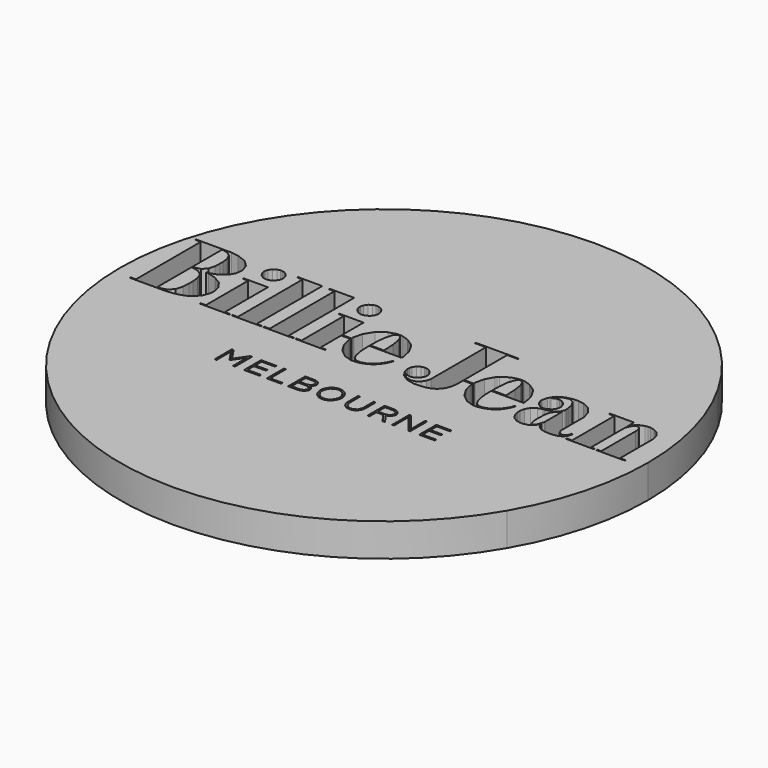
from build123d import *
from build123d import SkipClean  # not in build123d's __all__

# Parameters (mm, degrees)
F1_DEPTH = 5
F3_DEPTH = 50
F5_DEPTH = 25


with BuildPart() as f1:
    # F0 (on Top) → F1 (new body)
    with BuildSketch(Plane.XY):
        with BuildLine():
            Line((34.6410161514, -20), (40, -20))
            Line((40, -20), (40, 0))
            ThreePointArc((40, 0), (38.6370330516, -10.3527618041), (34.6410161514, -20))
        make_face()
        with BuildLine():
            ThreePointArc((-34.6410161514, -20), (0, -40), (34.6410161514, -20))
            Line((34.6410161514, -20), (-34.6410161514, -20))
        make_face()
        with BuildLine():
            Line((-34.6410161514, -20), (34.6410161514, -20))
            ThreePointArc((34.6410161514, -20), (38.6370330516, -10.3527618041), (40, 0))
            ThreePointArc((40, 0), (38.6370330516, 10.3527618041), (34.6410161514, 20))
            Line((34.6410161514, 20), (-34.6410161514, 20))
            ThreePointArc((-34.6410161514, 20), (-38.6370330532, 10.352761798), (-40, -1.26e-08))
            ThreePointArc((-40, -1.26e-08), (-38.6370330499, -10.3527618102), (-34.6410161514, -20))
        make_face()
        with BuildLine():
            ThreePointArc((34.6410161514, 20), (38.6370330516, 10.3527618041), (40, 0))
            Line((40, 0), (40, 20))
            Line((40, 20), (34.6410161514, 20))
        make_face()
        with BuildLine():
            Line((-40, -20), (-34.6410161514, -20))
            ThreePointArc((-34.6410161514, -20), (-38.6370330499, -10.3527618102), (-40, -1.26e-08))
            Line((-40, -1.26e-08), (-40, -20))
        make_face()
        with BuildLine():
            Line((-34.6410161514, 20), (34.6410161514, 20))
            ThreePointArc((34.6410161514, 20), (0, 40), (-34.6410161514, 20))
        make_face()
        with BuildLine():
            Line((-40, 20), (-40, -1.26e-08))
            ThreePointArc((-40, -1.26e-08), (-38.6370330532, 10.352761798), (-34.6410161514, 20))
            Line((-34.6410161514, 20), (-40, 20))
        make_face()
    extrude(amount=F1_DEPTH)

    # F2 (on face) → F3 (cut)
    with BuildSketch(Plane.XY.offset(5)):
        Polygon((-30.8900436095, 5.3960228478), (-31.2979021822, 5.4461403697), (-30.9122151654, 5.5068806273), (-29.7861507128, 5.9029180019), (-28.8714514615, 6.6135517779), (-28.4207478551, 7.4603744723), (-28.2995941933, 8.1075442124), (-28.2995941933, 8.3219055699), (-28.2995941933, 8.6691873117), (-28.6749036146, 9.7093982701), (-29.6517050126, 10.6270392021), (-31.0141661897, 11.1355686232), (-32.1609313579, 11.2905516123), (-32.5421786159, 11.2905516123), (-37.5014980781, 11.2905516123), (-37.5014980781, 11.1399266686), (-36.6901934536, 11.1399266686), (-36.6901934536, -1.1312668693), (-37.5014980781, -1.1312668693), (-37.5014980781, -1.2834716044), (-32.3973553202, -1.2834716044), (-32.2407108263, -1.2834716044), (-31.7707773446, -1.2598292082), (-30.9846131944, -1.1682013039), (-30.120167654, -0.9687117763), (-29.4625658428, -0.7293188956), (-29.255667638, -0.6243989529), (-28.9704608052, -0.4766339765), (-27.9685734084, 0.5046071803), (-27.5370452016, 1.7119219416), (-27.5370452016, 2.1138699153), (-27.5370452016, 2.4286297434), (-27.7838467595, 3.3729092277), (-28.5079087629, 4.3600609836), (-29.687168607, 5.0574571967), align=None)
        Polygon((-33.4731388241, -1.1194456712), (-33.4731388241, 5.3486291042), (-33.1716982722, 5.347267215), (-32.2687657434, 5.1462523715), (-31.5506143391, 4.5683755531), (-31.2033325973, 3.6329755862), (-31.1132027711, 2.6739059853), (-31.1132027711, 2.3532627959), (-31.1132027711, 1.9926617779), (-31.173779602, 0.9080259943), (-31.4693367927, -0.1810495481), (-32.1771923147, -0.8697296704), (-33.1495267163, -1.1164767527), align=None, mode=Mode.SUBTRACT)
        Polygon((-33.1864611509, 5.5275813429), (-33.4731388241, 5.5142348289), (-33.4731388241, 11.1369305124), (-33.2426254609, 11.1355686232), (-32.5495600553, 10.9773171001), (-31.9141025622, 10.5061034426), (-31.5476454207, 9.6990479124), (-31.4294334396, 8.8241703008), (-31.4294334396, 8.5316365042), (-31.4294334396, 8.2213981481), (-31.4752473917, 7.2860526568), (-31.7205508715, 6.3580613671), (-32.3323387305, 5.7623710382), align=None, mode=Mode.SUBTRACT)
        Polygon((-23.2205646719, -1.1312668693), (-23.2205646719, 7.0289279789), (-26.9016149464, 7.0289279789), (-26.9016149464, 6.8780306574), (-26.0918084, 6.8780306574), (-26.0918084, -1.1312668693), (-26.9016149464, -1.1312668693), (-26.9016149464, -1.2834716044), (-22.4092600475, -1.2834716044), (-22.4092600475, -1.1312668693), align=None)
        Polygon((-18.3852588388, -1.1312668693), (-18.3852588388, 11.2905516123), (-22.0664453022, 11.2905516123), (-22.0664453022, 11.1399266686), (-21.2566659936, 11.1399266686), (-21.2566659936, -1.1312668693), (-22.0664453022, -1.1312668693), (-22.0664453022, -1.2834716044), (-17.5741176411, -1.2834716044), (-17.5741176411, -1.1312668693), align=None)
        Polygon((-13.5516417483, -1.1312668693), (-13.5516417483, 11.2905516123), (-17.2328282117, 11.2905516123), (-17.2328282117, 11.1399266686), (-16.4230489031, 11.1399266686), (-16.4230489031, -1.1312668693), (-17.2328282117, -1.1312668693), (-17.2328282117, -1.2834716044), (-12.7405005506, -1.2834716044), (-12.7405005506, -1.1312668693), align=None)
        Polygon((-4.475467473, 2.7891762858), (0.4262440767, 2.7891762858), (0.4262440767, 2.9532294569), (0.4202517643, 3.244319651), (0.1130095645, 4.6082789062), (-0.5428762664, 5.7890640662), (-0.7218285051, 5.9870827535), (-0.9024150109, 6.18646333), (-1.9630543071, 6.9047236854), (-3.0699978355, 7.22395051), (-3.4379802929, 7.22395051), (-3.8103207957, 7.22395051), (-4.9273423041, 6.8957352168), (-6.1437817229, 5.9930750659), (-6.9728998579, 4.6437697383), (-7.2918543047, 3.3921118652), (-7.3008427733, 2.9724320944), (-8.7163903908, 2.9724320944), (-8.7163903908, 7.0289279789), (-12.3975768541, 7.0289279789), (-12.3975768541, 6.8780306574), (-11.5877975455, 6.8780306574), (-11.5877975455, -1.1312668693), (-12.3975768541, -1.1312668693), (-12.3975768541, -1.2834716044), (-7.9049768152, -1.2834716044), (-7.9049768152, -1.1312668693), (-8.7163903908, -1.1312668693), (-8.7163903908, 2.7891762858), (-7.3038389295, 2.7891762858), (-7.2994808842, 2.3842866316), (-6.9993205081, 1.1695904309), (-6.2001639351, -0.1574071518), (-5.0188612573, -1.0662502796), (-3.9312565552, -1.4194426205), (-3.5651807427, -1.4312365809), (-3.4853740365, -1.4312365809), (-3.2413234948, -1.4164737021), (-2.8008885328, -1.3558696334), (-2.2839153987, -1.2228947735), (-1.7225446772, -0.9923541725), (-1.1549092655, -0.6347493107), (-0.6139668818, -0.1263833162), (-0.139757068, 0.5622423306), (0.1633994643, 1.2242566627), (0.235579591, 1.4533264234), (0.2549184174, 1.5183157753), (0.0983011613, 1.5183157753), (-0.0155527745, 1.1917619868), (-0.1040755714, 0.9671319849), (-0.7351750191, -0.0037588141), (-1.6024260512, -0.7396692534), (-1.808071318, -0.8475581145), (-1.9085787397, -0.8933720667), (-2.63882372, -1.1267998727), (-2.8809676168, -1.1267998727), (-3.0964184857, -1.1267998727), (-3.6877507692, -0.8386513593), (-3.7438606036, -0.7825142871), (-3.8871313457, -0.6391890694), (-4.1676805175, -0.0643628828), (-4.3869446761, 0.8784457612), (-4.4667513822, 1.8848273923), (-4.4768293622, 2.5646007595), align=None)
        Polygon((-3.6033136398, 7.0643370977), (-3.4630390539, 7.0716912993), (-3.4453344945, 7.0716912993), (-3.3287567804, 7.0656989869), (-2.9871949731, 6.8072124198), (-2.6666062593, 6.0549048348), (-2.4759417736, 4.7856513535), (-2.4108434706, 3.4261046192), (-2.4094815814, 2.9724320944), (-4.475467473, 2.9724320944), (-4.475467473, 3.3152468397), (-4.4414202434, 4.339360268), (-4.3025075467, 5.6545094148), (-3.9979891252, 6.6535913199), align=None, mode=Mode.SUBTRACT)
        Polygon((-10.013998405, 11.3542880261), (-10.1529111017, 11.3542880261), (-10.2931856876, 11.3542880261), (-10.711285667, 11.2417959796), (-11.1680632992, 10.9345537797), (-11.4755778768, 10.4777761475), (-11.5877975455, 10.0596761682), (-11.5877975455, 9.9194015823), (-11.5877975455, 9.7804888855), (-11.4755778768, 9.3607546391), (-11.1680632992, 8.903977007), (-10.711285667, 8.5967348071), (-10.2931856876, 8.4828808714), (-10.1529111017, 8.4828808714), (-10.013998405, 8.4828808714), (-9.5942641586, 8.5967348071), (-9.1374865264, 8.903977007), (-8.8305167044, 9.3607546391), (-8.7163903908, 9.7804888855), (-8.7163903908, 9.9194015823), (-8.7163903908, 10.0596761682), (-8.8305167044, 10.4777761475), (-9.1374865264, 10.9345537797), (-9.5942641586, 11.2417959796), align=None)
        Polygon((-24.5165656569, 11.3542880261), (-24.655423878, 11.3542880261), (-24.7958346529, 11.3542880261), (-25.2140435834, 11.2417959796), (-25.6706577888, 10.9345537797), (-25.9794797801, 10.4777761475), (-26.0918084, 10.0596761682), (-26.0918084, 9.9194015823), (-26.0918084, 9.7804888855), (-25.9794797801, 9.3607546391), (-25.6706577888, 8.903977007), (-25.2140435834, 8.5967348071), (-24.7958346529, 8.4828808714), (-24.655423878, 8.4828808714), (-24.5165656569, 8.4828808714), (-24.0968586483, 8.5967348071), (-23.6402716805, 8.903977007), (-23.3328932918, 9.3607546391), (-23.2190938316, 9.7804888855), (-23.2190938316, 9.9194015823), (-23.2190938316, 10.0596761682), (-23.3328932918, 10.4777761475), (-23.6402716805, 10.9345537797), (-24.0968586483, 11.2417959796), align=None)
        Polygon((14.0187152627, 2.7891762858), (18.9204268124, 2.7891762858), (18.9204268124, 2.9532294569), (18.9144345, 3.244319651), (18.6071923002, 4.6082789062), (17.9507617137, 5.7890640662), (17.7723542306, 5.9870827535), (17.5917677249, 6.18646333), (16.530583673, 6.9047236854), (15.4241849002, 7.22395051), (15.055930065, 7.22395051), (14.6863133406, 7.22395051), (13.5799145678, 6.9060855746), (12.5170962489, 6.188097597), (12.338416388, 5.9884446427), (12.1597365271, 5.7920602224), (11.5079363638, 4.6186565018), (11.1993322748, 3.2620514482), (11.1930675846, 2.9724320944), (9.7538230953, 2.9724320944), (9.7538230953, 11.1369305124), (11.4047051637, 11.1369305124), (11.4047051637, 11.2905516123), (4.8951472438, 11.2905516123), (4.8951472438, 11.1399266686), (6.539764622, 11.1399266686), (6.539764622, 0.9479021096), (6.539764622, 0.7321788629), (6.3932253458, 0.0819857289), (6.0124411301, -0.5224479286), (5.4815767263, -0.877083872), (5.0370560968, -0.9938522506), (4.8891549314, -0.9938522506), (4.6557271253, -0.9938522506), (3.9565332185, -0.7219102185), (3.3447725972, -0.1293522347), (3.2548879111, 0.0302339399), (3.3194414584, -0.0259031323), (3.9892185589, -0.3229311632), (4.2122960072, -0.3229311632), (4.3512087039, -0.3229311632), (4.7695810611, -0.2091589408), (5.2260863154, 0.0982194479), (5.5333285153, 0.5548608912), (5.647182451, 0.9730425839), (5.647182451, 1.1119552806), (5.647182451, 1.2523388177), (5.5333285153, 1.6705477482), (5.2260863154, 2.1271619537), (4.7695810611, 2.4360111827), (4.3512087039, 2.5483125648), (4.2122960072, 2.5483125648), (4.0720214212, 2.5483125648), (3.653649064, 2.4404237037), (3.1968714319, 2.1463645912), (2.8899016099, 1.7104511013), (2.7774095633, 1.311472046), (2.7774095633, 1.1769718703), (2.7774095633, 0.9464312693), (2.9473733334, 0.2504241831), (3.5013898533, -0.6007565567), (4.5031955368, -1.2243656139), (5.6411901386, -1.466727413), (6.020884843, -1.466727413), (6.1837667894, -1.466727413), (6.6743192733, -1.4445558571), (7.3258470588, -1.3617802325), (7.9495923049, -1.1918437002), (8.519951495, -0.9110766261), (9.0118658681, -0.491424093), (9.3978252627, 0.0908380085), (9.6535880514, 0.8622392799), (9.7505545613, 1.6025622402), (9.7538230953, 1.8478657199), (9.7538230953, 2.7891762858), (11.1900714284, 2.7891762858), (11.1947018516, 2.3842866316), (11.4962241168, 1.1681195906), (12.2956530676, -0.1589324677), (13.476138612, -1.0662502796), (14.563743314, -1.4194426205), (14.9303638823, -1.4312365809), (15.0101705884, -1.4312365809), (15.2539487523, -1.4164737021), (15.6930218251, -1.3558696334), (16.210267337, -1.2228947735), (16.7716380585, -0.9923541725), (17.3390010924, -0.6347493107), (17.8799434762, -0.1263833162), (18.3544256677, 0.5622423306), (18.6570374443, 1.2242566627), (18.7297623267, 1.4533264234), (18.7504630423, 1.5183157753), (18.5935734084, 1.5183157753), (18.4799918505, 1.1917619868), (18.3911966757, 0.9671319849), (17.760097228, -0.0037588141), (16.8912119288, -0.7396692534), (16.6861114178, -0.8475581145), (16.585603996, -0.8933720667), (15.8553590158, -1.1267998727), (15.6132151189, -1.1267998727), (15.3972194944, -1.1267998727), (14.8064319666, -0.8386513593), (14.7500497544, -0.7825142871), (14.6065066344, -0.6391890694), (14.3259574626, -0.0643628828), (14.1088723267, 0.8784457612), (14.0287932427, 1.8848273923), (14.0187152627, 2.5646007595), align=None)
        Polygon((14.8903243403, 7.0643370977), (15.0311436819, 7.0716912993), (15.0483034856, 7.0716912993), (15.1654259554, 7.0656989869), (15.5064430069, 6.8072124198), (15.8273040986, 6.0549048348), (16.0179685843, 4.7856513535), (16.0830668873, 3.4261046192), (16.0847011543, 2.9724320944), (14.0187152627, 2.9724320944), (14.0187152627, 3.3152468397), (14.0527624923, 4.339360268), (14.1916751891, 5.6545094148), (14.4956488549, 6.6535913199), align=None, mode=Mode.SUBTRACT)
        Polygon((28.2934929298, 0.1957307135), (28.2934929298, 0.1395936413), (28.2934929298, -0.0126110938), (28.0881200409, -0.4707233774), (27.6787361523, -0.6997386625), (27.5430919896, -0.6997386625), (27.4098992275, -0.6997386625), (27.0152237421, -0.4810464974), (26.7921462938, -0.058425046), (26.7921462938, 0.0435532161), (26.7921462938, 3.9048631428), (26.7921462938, 4.3245701515), (26.4789117815, 5.5806950211), (25.6764866745, 6.5928510623), (24.5842515493, 7.0923920149), (23.6979340686, 7.22395051), (23.4021317379, 7.22395051), (23.0385073259, 7.22395051), (21.9525368909, 7.0008730618), (21.0229113341, 6.4893474844), (20.879640592, 6.3447148531), (20.7630628779, 6.2294990282), (20.3446905207, 5.5392935899), (20.1586564582, 4.7442499223), (20.1600183474, 4.5743133899), (20.1660106598, 4.439840452), (20.2902149533, 4.036421638), (20.6004533094, 3.6019789884), (21.0498767399, 3.3123051591), (21.4576263615, 3.205914376), (21.5935429021, 3.205914376), (21.7321832209, 3.205914376), (22.1521898452, 3.3197138362), (22.6086950995, 3.627092225), (22.9159372993, 4.0837064304), (23.0297912351, 4.5019153609), (23.0297912351, 4.6407735821), (23.0297912351, 4.7811843569), (22.9159372993, 5.1993660497), (22.6086950995, 5.655871304), (22.1521898452, 5.9647477709), (21.7321832209, 6.0772398174), (21.5935429021, 6.0772398174), (21.3454066928, 6.0772398174), (20.6669135015, 5.7653671944), (20.6018151985, 5.7062612038), (20.6538393654, 5.8111266709), (21.0438844275, 6.2839745955), (21.5818306551, 6.6726577685), (21.708758727, 6.7347599153), (21.7812112316, 6.7688071449), (22.3308697061, 6.9327786026), (22.5158142572, 6.9327786026), (22.7135605667, 6.9327786026), (23.3119746739, 6.5944853294), (23.7319812982, 5.8274693412), (23.8943184889, 5.0160557655), (23.922373406, 4.6570617767), (23.922373406, 4.5373517175), (23.922373406, 4.3940264998), (23.7864568655, 3.9625255309), (23.3950499141, 3.5014443289), (22.7685808897, 3.171921622), (22.1432013766, 3.0153043659), (21.9334704423, 2.99313281), (21.7057625708, 2.9694904138), (21.0392540043, 2.7655338896), (20.3863643297, 2.3059780035), (19.9840622648, 1.6247337961), (19.8484181022, 0.9612213858), (19.8484181022, 0.7395330645), (19.8484181022, 0.5164283784), (19.9963192675, -0.1544654712), (20.4157811361, -0.8401221996), (21.0749355009, -1.2760901651), (21.722105241, -1.4312365809), (21.9378284877, -1.4312365809), (22.1551860014, -1.4312365809), (22.8110718322, -1.2775610054), (23.4051278941, -0.9096057857), (23.7687523061, -0.4692525371), (23.9150192045, -0.1899563033), (23.9520625902, -0.0924178), (23.9771213512, -0.2800861295), (24.2345184069, -0.8209467999), (24.776550302, -1.2243656139), (25.5035267482, -1.3943021462), (26.1346261959, -1.4312365809), (26.3459913972, -1.4312365809), (26.5734268909, -1.4312365809), (27.2609085508, -1.3322272372), (27.9167943816, -1.0366972844), (28.311469867, -0.5475611652), (28.4443902513, -0.034755412), (28.4443902513, 0.1351538826), (28.4443902513, 0.1794969944), align=None)
        Polygon((23.922373406, 3.8650142653), (23.922373406, 0.6257880799), (23.9237352952, 0.531218495), (23.650540325, -0.3835352319), (23.5944304906, -0.4736650581), (23.54540248, -0.5357127293), (23.2267204111, -0.8519706355), (23.1213101882, -0.8519706355), (23.0888972257, -0.8519706355), (22.9957440055, -0.7943354852), (22.8655473996, -0.5564134449), (22.7623161994, -0.0436621672), (22.7228214131, 0.6213210834), (22.7228214131, 0.8430094047), (22.7228214131, 1.1163678016), (22.7653123556, 1.9321121848), (22.8818900698, 2.6148272326), (23.0491300615, 2.9960744906), (23.1894046474, 3.1497500661), (23.2455144818, 3.1837428201), (23.3119746739, 3.2295567723), (23.8826062419, 3.7866511617), align=None, mode=Mode.SUBTRACT)
        Polygon((37.5014980781, -1.1312668693), (36.6900845025, -1.1312668693), (36.6900845025, 4.9629420874), (36.6900845025, 5.2274209668), (36.4877077698, 6.019495716), (35.9617461671, 6.7184172451), (35.2271431415, 7.1057385289), (34.6093902078, 7.22395051), (34.4040173189, 7.22395051), (34.2547542643, 7.22395051), (33.811595524, 7.1485018493), (33.2069167265, 6.898731373), (32.6678809876, 6.4495803202), (32.3393933165, 5.9516736347), (32.2732055022, 5.7697252398), (32.2732055022, 7.0289279789), (28.5920190388, 7.0289279789), (28.5920190388, 6.8780306574), (29.4020707253, 6.8780306574), (29.4020707253, -1.1312668693), (28.5920190388, -1.1312668693), (28.5920190388, -1.2834716044), (32.8626311408, -1.2834716044), (32.8626311408, -1.1312668693), (32.2732055022, -1.1312668693), (32.2732055022, 5.0116977202), (32.2732055022, 5.333920701), (32.6842236578, 6.2058021564), (32.764030364, 6.3003172657), (32.7920852811, 6.3343644953), (33.1107673501, 6.511682467), (33.2191737291, 6.511682467), (33.2690188732, 6.511682467), (33.4199161948, 6.471642925), (33.6152111037, 6.2943249533), (33.7612056242, 5.8925676441), (33.8189497256, 5.358979462), (33.8189497256, 5.1802996011), (33.8189497256, -1.1312668693), (33.2292517091, -1.1312668693), (33.2292517091, -1.2834716044), (37.5014980781, -1.2834716044), align=None)
        Polygon((-13.8294671418, -8.057481166), (-15.0870356139, -9.9105493026), (-16.3446040861, -8.057481166), (-16.6164371672, -8.057481166), (-16.6164371672, -11.2996217943), (-16.3239033705, -11.2996217943), (-16.3239033705, -8.6145483176), (-15.1284370451, -10.3553423099), (-15.1180866873, -10.3701051887), (-15.0649730092, -10.3701051887), (-13.859156326, -8.6145483176), (-13.859156326, -11.2996217943), (-13.5559997937, -11.2996217943), (-13.5559997937, -8.057481166), align=None)
        Polygon((-11.8716152514, -11.0159130396), (-11.8716152514, -9.807127438), (-10.0524036799, -9.807127438), (-10.0524036799, -9.5233914454), (-11.8716152514, -9.5233914454), (-11.8716152514, -8.3411899207), (-9.8483926802, -8.3411899207), (-9.8483926802, -8.057481166), (-12.1744994059, -8.057481166), (-12.1744994059, -11.2996217943), (-9.8263300755, -11.2996217943), (-9.8263300755, -11.0159130396), align=None)
        Polygon((-8.4282146395, -11.0159130396), (-8.4282146395, -8.057481166), (-8.7297369048, -8.057481166), (-8.7297369048, -11.2996217943), (-6.5635159693, -11.2996217943), (-6.5635159693, -11.0159130396), align=None)
        Polygon((-3.4573191193, -9.6607788263), (-3.5635464756, -9.6268133101), (-3.5058023743, -9.5972603148), (-3.2372378273, -9.3637780331), (-3.0863405057, -9.0002353345), (-3.0863405057, -8.880552513), (-3.0863405057, -8.8717002333), (-3.0863405057, -8.7224371788), (-3.376150524, -8.2776441714), (-3.956587694, -8.057481166), (-4.1488864468, -8.057481166), (-5.4933434488, -8.057481166), (-5.4933434488, -11.2996217943), (-4.0807919876, -11.2996217943), (-3.8680648971, -11.2996217943), (-3.2282493586, -11.0542910768), (-2.9087501562, -10.5622405147), (-2.9087501562, -10.3996854218), (-2.9087501562, -10.3908059043), (-2.9087501562, -10.2725939231), (-3.0759901479, -9.9223432629), align=None)
        Polygon((-5.1907316722, -11.0159130396), (-5.1907316722, -9.807127438), (-4.1488864468, -9.807127438), (-3.9759265204, -9.807127438), (-3.4573191193, -9.9563632547), (-3.2162647338, -10.2814734406), (-3.2162647338, -10.3908059043), (-3.2162647338, -10.3996854218), (-3.2162647338, -10.5119595661), (-3.4466963837, -10.8489181879), (-3.916548152, -11.0159130396), (-4.0720758968, -11.0159130396), align=None, mode=Mode.SUBTRACT)
        Polygon((-5.1907316722, -8.3411899207), (-4.1529721143, -8.3411899207), (-4.0143317954, -8.3411899207), (-3.5975937052, -8.4889548971), (-3.3922208163, -8.7918935271), (-3.3922208163, -8.8938445514), (-3.3922208163, -8.9026968311), (-3.3922208163, -9.015025451), (-3.6033136398, -9.3563965938), (-4.033398244, -9.5233914454), (-4.176941364, -9.5233914454), (-5.1907316722, -9.5233914454), align=None, mode=Mode.SUBTRACT)
        Polygon((1.3528734772, -9.6740981025), (1.3485154318, -9.6563663053), (1.3471535427, -9.490842294), (1.2215873599, -8.9987644941), (0.8783912857, -8.4741647806), (0.3641419299, -8.1269102766), (-0.1174220854, -8.0027604586), (-0.2770354977, -8.0027604586), (-0.4497230462, -8.0027604586), (-0.9642447798, -8.1475837544), (-1.4784941355, -8.5318271686), (-1.8007171164, -9.0682208425), (-1.9115748959, -9.5248622858), (-1.9115748959, -9.6785378612), (-1.9115748959, -9.6874173787), (-1.9115748959, -9.8514160742), (-1.7887324916, -10.3479336328), (-1.4474430621, -10.8770003428), (-0.9318318172, -11.2272237653), (-0.448361157, -11.3542880261), (-0.2860239663, -11.3542880261), (-0.1163325741, -11.3542880261), (0.3981891595, -11.2094919681), (0.9108042482, -10.8297155504), (1.2332996069, -10.2962363194), (1.3471535427, -9.8410929542), (1.3485154318, -9.6903590594), (1.3485154318, -9.688888219), (1.3528734772, -9.6770670209), align=None)
        Polygon((-0.1471112696, -11.0749917923), (-0.2770354977, -11.0749917923), (-0.4072321037, -11.0749917923), (-0.797004788, -10.9656593287), (-1.2170114123, -10.6701021381), (-1.4978329619, -10.226779971), (-1.599429895, -9.8144816396), (-1.599429895, -9.6785378612), (-1.599429895, -9.6696855816), (-1.599429895, -9.5307728848), (-1.5008291181, -9.1184473156), (-1.2243656139, -8.6781213047), (-0.8076275237, -8.3870038728), (-0.4173100836, -8.2820566924), (-0.2860239663, -8.2820566924), (-0.1574616274, -8.2820566924), (0.2325834348, -8.3899455535), (0.6539519482, -8.6854755063), (0.9347734979, -9.1288249112), (1.038004698, -9.5410960048), (1.038004698, -9.6785378612), (1.038004698, -9.6874173787), (1.038004698, -9.8248319974), (0.9377696541, -10.2371303288), (0.6613061498, -10.6774835774), (0.2432061704, -10.9686282471), align=None, mode=Mode.SUBTRACT)
        Polygon((4.8861587752, -8.057481166), (4.8861587752, -9.9459856591), (4.8861587752, -10.1528838639), (4.6170494725, -10.7765201589), (4.0496864386, -11.0705792714), (3.8620181091, -11.0705792714), (3.6683574672, -11.0705792714), (3.0922783425, -10.7691114817), (2.8201728837, -10.1351520667), (2.8201728837, -9.9238685788), (2.8201728837, -8.057481166), (2.5172887292, -8.057481166), (2.5172887292, -9.9459856591), (2.5172887292, -10.0908361927), (2.6090800602, -10.529718601), (2.8765550959, -10.9715699277), (3.2960169644, -11.2508661615), (3.7130274324, -11.3498755052), (3.8533020184, -11.3498755052), (3.9922147151, -11.3498755052), (4.4086804274, -11.2493953212), (4.8286870517, -10.9641884884), (5.0945278203, -10.5149557223), (5.1876810405, -10.0671937965), (5.1876810405, -9.9194015823), (5.1876810405, -8.057481166), align=None)
        Polygon((9.0666138133, -9.155408988), (9.0666138133, -9.0032314907), (9.0666138133, -8.9943247354), (9.0666138133, -8.8243882031), (8.7443908324, -8.3145513683), (8.1108399842, -8.057481166), (7.8992024051, -8.057481166), (6.5324104204, -8.057481166), (6.5324104204, -11.2996217943), (6.8339326856, -11.2996217943), (6.8339326856, -9.9844181719), (7.8240261221, -9.9844181719), (8.8348202742, -11.2996217943), (9.217238757, -11.2996217943), (8.1636812845, -9.9341916988), (8.3039558704, -9.9105493026), (8.8271936948, -9.61649019), align=None)
        Polygon((6.8339326856, -9.7051219381), (6.8339326856, -8.3411899207), (7.8844940019, -8.3411899207), (8.0457416812, -8.3411899207), (8.5303018528, -8.5170370521), (8.7637296588, -8.880552513), (8.7637296588, -9.0032314907), (8.7637296588, -9.0120837703), (8.7637296588, -9.1376771909), (8.519951495, -9.5159827683), (8.0323951672, -9.7051219381), (7.8711474879, -9.7051219381), align=None, mode=Mode.SUBTRACT)
        Polygon((12.698772266, -8.057481166), (12.698772266, -10.7587883617), (10.5665985601, -8.0707459666), (10.5559758245, -8.057481166), (10.2860493883, -8.057481166), (10.2860493883, -11.2996217943), (10.5783108071, -11.2996217943), (10.5783108071, -8.539208608), (12.7567887452, -11.2878005962), (12.765504836, -11.2996217943), (12.9915784405, -11.2996217943), (12.9915784405, -8.057481166), align=None)
        Polygon((16.7198862695, -11.0159130396), (14.6732392044, -11.0159130396), (14.6732392044, -9.807127438), (16.4938126651, -9.807127438), (16.4938126651, -9.5233914454), (14.6732392044, -9.5233914454), (14.6732392044, -8.3411899207), (16.6978236648, -8.3411899207), (16.6978236648, -8.057481166), (14.3717169391, -8.057481166), (14.3717169391, -11.2996217943), (16.7198862695, -11.2996217943), align=None)
    extrude(amount=-F3_DEPTH, mode=Mode.SUBTRACT)

    # F4 (on face) → F5 (cut)
    with BuildSketch(Plane.XY.offset(5)):
        with BuildLine():
            ThreePointArc((-40, -1.26e-08), (-38.6370330532, 10.352761798), (-34.6410161514, 20))
            Line((-34.6410161514, 20), (-40, 20))
            Line((-40, 20), (-40, -1.26e-08))
        make_face()
        with BuildLine():
            Line((40, -20), (40, 0))
            ThreePointArc((40, 0), (38.6370330516, -10.3527618041), (34.6410161514, -20))
            Line((34.6410161514, -20), (40, -20))
        make_face()
        with BuildLine():
            ThreePointArc((34.6410161514, 20), (38.6370330516, 10.3527618041), (40, 0))
            Line((40, 0), (40, 20))
            Line((40, 20), (34.6410161514, 20))
        make_face()
        with BuildLine():
            Line((-40, -20), (-34.6410161514, -20))
            ThreePointArc((-34.6410161514, -20), (-38.6370330499, -10.3527618102), (-40, -1.26e-08))
            Line((-40, -1.26e-08), (-40, -20))
        make_face()
    with SkipClean():  # cleaning this boolean's faces spoils the solid; the shape is the same uncleaned
        extrude(amount=-F5_DEPTH, mode=Mode.SUBTRACT)


solid = f1.part
